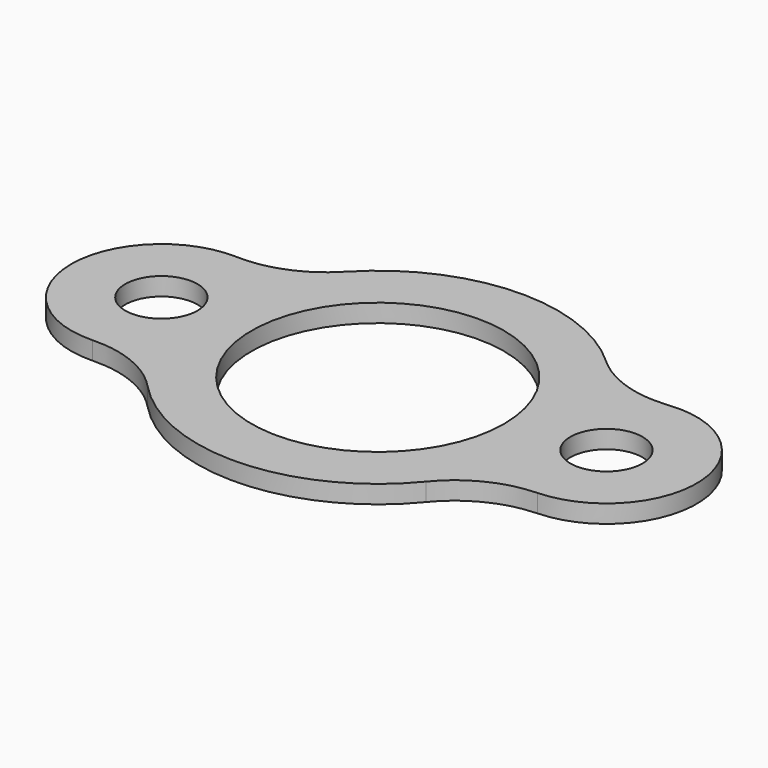
from build123d import *

# Parameters (mm, degrees)
F0_R     = 63.5
F0_R_2   = 44.45
F1_DEPTH = 6.35
F2_R     = 31.75
F2_R_2   = 12.7
F3_DEPTH = 6.35
F4_R     = 31.75
F4_R_2   = 12.7
F5_DEPTH = 6.35
F8_R     = 38.1


# Not quite as in the source:
# - two fillets or chamfers of one size are made in one step


with BuildPart() as f1:
    # F0 (on Top) → F1 (new body)
    with BuildSketch(Plane.XY):
        Circle(F0_R)
        Circle(F0_R_2, mode=Mode.SUBTRACT)
    extrude(amount=-F1_DEPTH)

    # F2 (on Top) → F3 (join)
    with BuildSketch(Plane.XY):
        with Locations((-76.2, 0)):
            Circle(F2_R)
        with Locations((-76.2, 0)):
            Circle(F2_R_2, mode=Mode.SUBTRACT)
    extrude(amount=-F3_DEPTH)

    # F4 (on Top) → F5 (join)
    with BuildSketch(Plane.XY):
        with Locations((76.2, 5.3983563557)):
            Circle(F4_R)
        with Locations((76.2, 5.3983563557)):
            Circle(F4_R_2, mode=Mode.SUBTRACT)
    extrude(amount=-F5_DEPTH)

    # F6: union 

    # F7: union 

    # F8
    f8_edges = [f1.edges().sort_by_distance(p)[0] for p in [
        (-57.94375, 25.976371, -3.175),
        (56.016218, 29.907078, -3.175),
        (59.673087, -21.711119, -3.175),
        (-57.94375, -25.976371, -3.175),
    ]]
    fillet(f8_edges, radius=F8_R)


solid = f1.part
